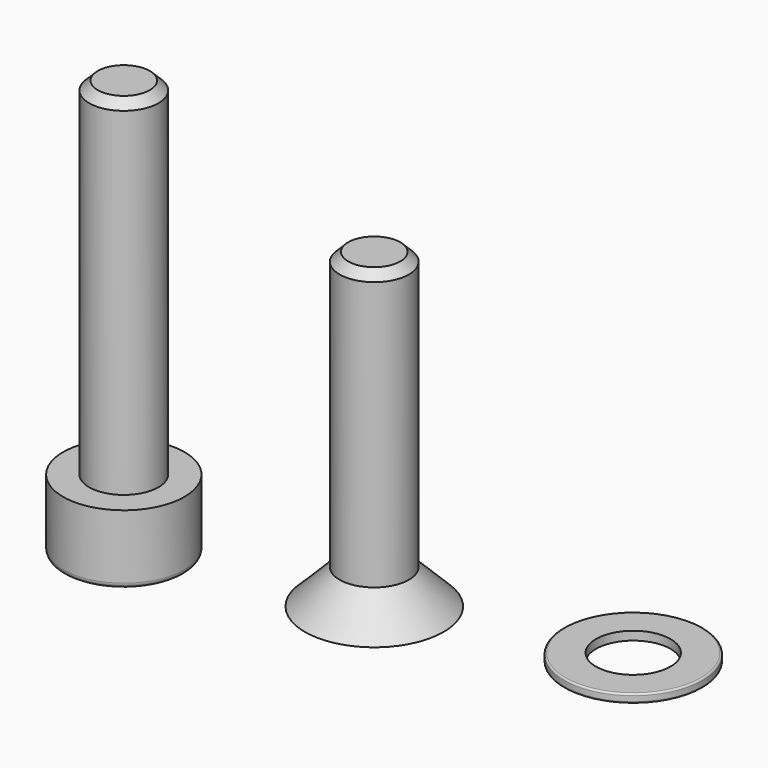
from build123d import *

# Parameters (mm, degrees)
F0_R      = 2
F1_DEPTH  = 20
F2_SIZE   = 0.5
F3_R      = 3.5
F4_DEPTH  = 4
F5_R      = 0.3
F7_DEPTH  = 2.5
F8_R      = 0.2
F9_R      = 2
F10_DEPTH = 16
F11_SIZE  = 0.5
F12_R     = 4
F13_DEPTH = 2
F15_DEPTH = 2.5
F16_R     = 0.2
F17_SIZE  = 1.99999
F18_R     = 4
F18_R_2   = 2.15
F19_DEPTH = 0.5
F20_R     = 0.1


# Not quite as in the source:
# - a fillet or chamfer is up to 0.001 mm smaller than in the source, because OpenCascade refuses the exact size


with BuildPart() as f1:
    # F0 (on Top) → F1 (new body)
    with BuildSketch(Plane.XY):
        Circle(F0_R)
    extrude(amount=F1_DEPTH)

    # F2
    f2_edges = [f1.edges().sort_by_distance(p)[0] for p in [
        (-2, 0, 20),
    ]]
    chamfer(f2_edges, length=F2_SIZE)

    # F3 (on face) → F4 (join)
    with BuildSketch(Plane(origin=(0, 0, 0), x_dir=(1, 0, 0), z_dir=(0, 0, -1))):
        Circle(F3_R)
    extrude(amount=F4_DEPTH)

    # F5
    f5_edges = [f1.edges().sort_by_distance(p)[0] for p in [
        (-3.5, 0, -4),
    ]]
    fillet(f5_edges, radius=F5_R)

    # F6 (on face) → F7 (cut)
    with BuildSketch(Plane(origin=(0, 0, -4), x_dir=(1, 0, 0), z_dir=(0, 0, -1))):
        Polygon((1.6874600466, 0.3904850718), (0.5055600313, 1.6566258041), (-1.1819000152, 1.2661407323), (-1.6874600466, -0.3904850718), (-0.5055600313, -1.6566258041), (1.1819000152, -1.2661407323), align=None)
    extrude(amount=-F7_DEPTH, mode=Mode.SUBTRACT)

    # F8
    f8_edges = [f1.edges().sort_by_distance(p)[0] for p in [
        (0.33817, 1.461383, -1.5),
        (1.43468, 0.437828, -1.5),
        (1.09651, -1.023555, -1.5),
        (-0.33817, -1.461383, -1.5),
        (-1.43468, -0.437828, -1.5),
        (-1.09651, 1.023555, -1.5),
    ]]
    fillet(f8_edges, radius=F8_R)


with BuildPart() as f10:
    # F9 (on Top) → F10 (new body)
    with BuildSketch(Plane.XY):
        with Locations((14.4443198481, 0)):
            Circle(F9_R)
    extrude(amount=F10_DEPTH)

    # F11
    f11_edges = [f10.edges().sort_by_distance(p)[0] for p in [
        (12.44432, 0, 16),
    ]]
    chamfer(f11_edges, length=F11_SIZE)

    # F12 (on face) → F13 (join)
    with BuildSketch(Plane(origin=(0, 0, 0), x_dir=(1, 0, 0), z_dir=(0, 0, -1))):
        with Locations((14.4443198481, 0)):
            Circle(F12_R)
    extrude(amount=F13_DEPTH)

    # F14 (on face) → F15 (cut)
    with BuildSketch(Plane(origin=(0, 0, -2), x_dir=(1, 0, 0), z_dir=(0, 0, -1))):
        Polygon((14.9357198231, -1.3571512067), (15.8653472574, -0.2530107417), (15.3739472825, 1.1041404651), (13.9529198732, 1.3571512067), (13.0232924389, 0.2530107417), (13.5146924138, -1.1041404651), align=None)
    extrude(amount=-F15_DEPTH, mode=Mode.SUBTRACT)

    # F16
    f16_edges = [f10.edges().sort_by_distance(p)[0] for p in [
        (14.225206, 1.230646, 0.5),
        (15.400534, 0.805081, 0.5),
        (15.619647, -0.425565, 0.5),
        (14.663434, -1.230646, 0.5),
        (13.488106, -0.805081, 0.5),
        (13.268992, 0.425565, 0.5),
    ]]
    fillet(f16_edges, radius=F16_R)

    # F17 (size 2 in the source; OpenCascade refuses exactly that, so slightly less here)
    f17_edges = [f10.edges().sort_by_distance(p)[0] for p in [
        (10.44432, 0, 0),
    ]]
    chamfer(f17_edges, length=F17_SIZE)


with BuildPart() as f19:
    # F18 (on Top) → F19 (new body)
    with BuildSketch(Plane.XY):
        with Locations((29.3805521813, 0)):
            Circle(F18_R)
        with Locations((29.3805521813, 0)):
            Circle(F18_R_2, mode=Mode.SUBTRACT)
    extrude(amount=F19_DEPTH)

    # F20
    f20_edges = [f19.edges().sort_by_distance(p)[0] for p in [
        (25.380552, 0, 0),
        (25.380552, 0, 0.5),
    ]]
    fillet(f20_edges, radius=F20_R)


solid = Compound([f1.part, f10.part, f19.part])
